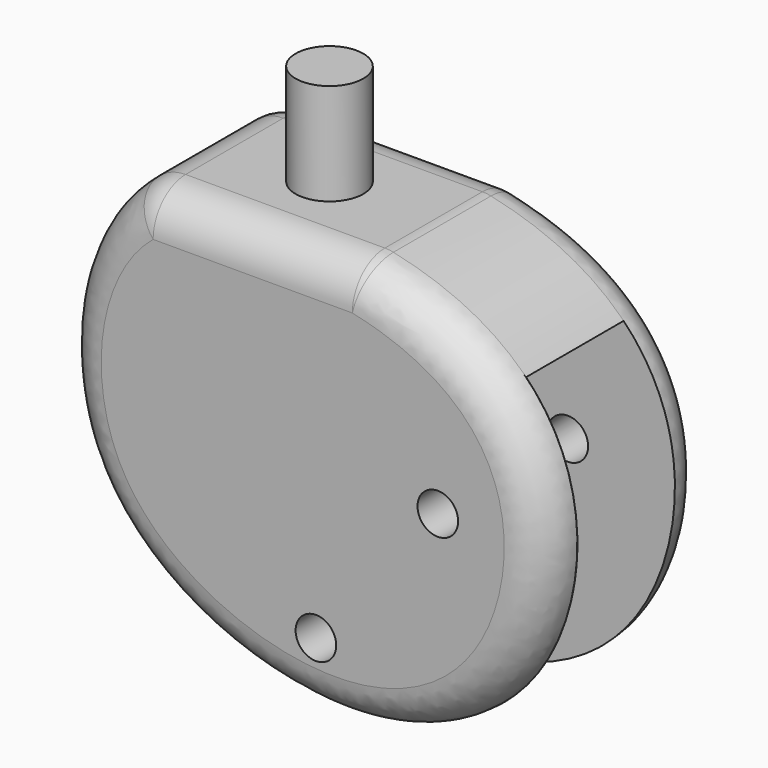
from build123d import *

# Parameters (mm, degrees)
F0_R     = 1.5
F1_DEPTH = 15
F2_R     = 2.5
F3_DEPTH = 7.5
F4_W     = 9
F4_H     = 26
F5_DEPTH = 25
F6_DEPTH = 25
F7_R     = 2.99999


# Not quite as in the source:
# - a fillet or chamfer is up to 0.001 mm smaller than in the source, because OpenCascade refuses the exact size


with BuildPart() as f1:
    # F0 (on Front) → F1 (new body)
    with BuildSketch(Plane.XZ):
        with BuildLine():
            Line((0, 20), (-16, 20))
            add(Edge.make_bspline(
                [(-16, 20), (-21.9968855381, 16.0502213985), (-25.0508954103, -3.343971526), (0.5714094097, -13.7693570255), (16.8200319307, -1.4098083557), (13.6831020936, 17.2049123794), (0, 20)],
                knots=[0, 0, 0, 0, 0.2484326246, 0.5085550507, 0.7313335966, 1, 1, 1, 1], degree=3))
        make_face()
        with Locations((-3, -5)):
            Circle(F0_R, mode=Mode.SUBTRACT)
        with Locations((6, 6)):
            Circle(F0_R, mode=Mode.SUBTRACT)
    extrude(amount=F1_DEPTH)

    # F2 (on face) → F3 (join)
    with BuildSketch(Plane.XY.offset(20)):
        with Locations((-8, -7.5)):
            Circle(F2_R)
    extrude(amount=F3_DEPTH)

    # F4 (on Right) → F5 (cut)
    with BuildSketch(Plane.YZ):
        with Locations((-7.5, 2)):
            Rectangle(F4_W, F4_H)
    extrude(amount=-F5_DEPTH, mode=Mode.SUBTRACT)

    # F4 (on Right) → F6 (cut)
    with BuildSketch(Plane.YZ):
        with Locations((-7.5, 2)):
            Rectangle(F4_W, F4_H)
    extrude(amount=F6_DEPTH, mode=Mode.SUBTRACT)

    # F7 (radius 3 in the source; OpenCascade refuses exactly that, so slightly less here)
    f7_edges = [f1.edges().sort_by_distance(p)[0] for p in [
        (-8, -15, 20),
        (-8, 0, 20),
        (-0.375905, 0, -10.026879),
        (-0.375905, -15, -10.026879),
        (-16, -7.5, 20),
        (0, -7.5, 20),
    ]]
    fillet(f7_edges, radius=F7_R)


solid = f1.part
